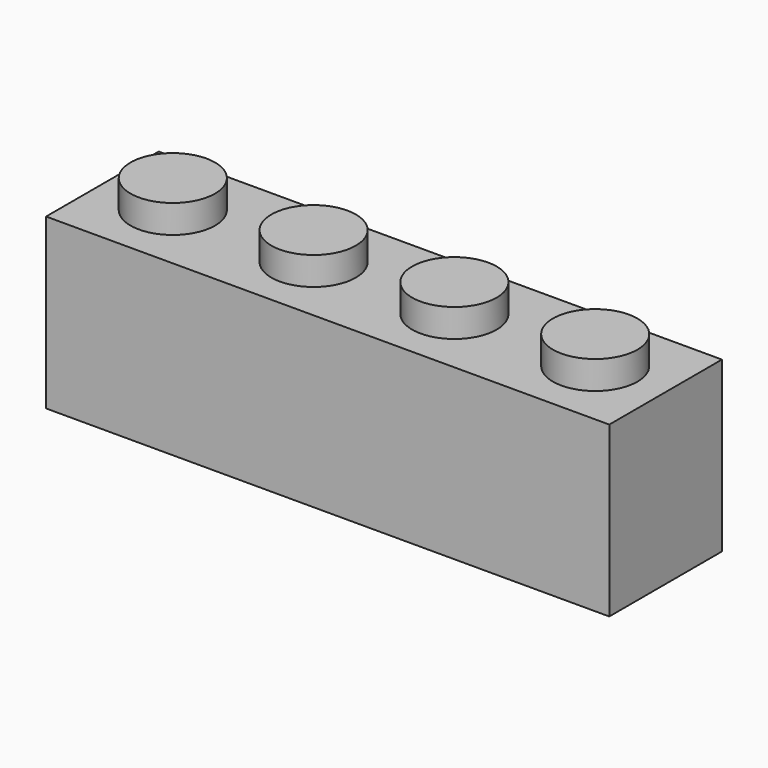
from build123d import *

# Parameters (mm, degrees)
F0_W     = 31.75
F0_H     = 7.9375
F0_R     = 2.38125
F1_DEPTH = 9.525
F2_DEPTH = 11.1125
F3_T     = -1.5875
F4_R     = 1.5875
F4_R_2   = 0.79375
F5_DEPTH = 7.9375


# Not quite as in the source:
# - a feature names something its author has since deleted; it is built from what else it names


with BuildPart() as f1:
    # F0 (on Top) → F1 (new body)
    with BuildSketch(Plane.XY):
        Rectangle(F0_W, F0_H)
        with Locations((-11.90625, 0)):
            Circle(F0_R, mode=Mode.SUBTRACT)
        with Locations((-3.96875, 0)):
            Circle(F0_R, mode=Mode.SUBTRACT)
        with Locations((3.96875, 0)):
            Circle(F0_R, mode=Mode.SUBTRACT)
        with Locations((11.90625, 0)):
            Circle(F0_R, mode=Mode.SUBTRACT)
    extrude(amount=F1_DEPTH)

    # F0 (on Top) → F2 (join)
    with BuildSketch(Plane.XY):
        with Locations((-11.90625, 0)):
            Circle(F0_R)
        with Locations((-3.96875, 0)):
            Circle(F0_R)
        with Locations((3.96875, 0)):
            Circle(F0_R)
        with Locations((11.90625, 0)):
            Circle(F0_R)
    extrude(amount=F2_DEPTH)

    # F3
    f3_openings = [f1.faces().sort_by_distance(p)[0] for p in [
        (0, 0, 0),
    ]]
    offset(amount=F3_T, openings=f3_openings, kind=Kind.INTERSECTION)

    # F4 (on face) → F5 (join)
    with BuildSketch(Plane(origin=(0, 0, 7.9375), x_dir=(1, 0, 0), z_dir=(0, 0, -1))):
        with Locations((-7.9375, 0)):
            Circle(F4_R)
        with Locations((-7.9375, 0)):
            Circle(F4_R_2, mode=Mode.SUBTRACT)
        Circle(F4_R)
        Circle(F4_R_2, mode=Mode.SUBTRACT)
        with Locations((7.9375, 0)):
            Circle(F4_R)
        with Locations((7.9375, 0)):
            Circle(F4_R_2, mode=Mode.SUBTRACT)
    extrude(amount=F5_DEPTH)


solid = f1.part
